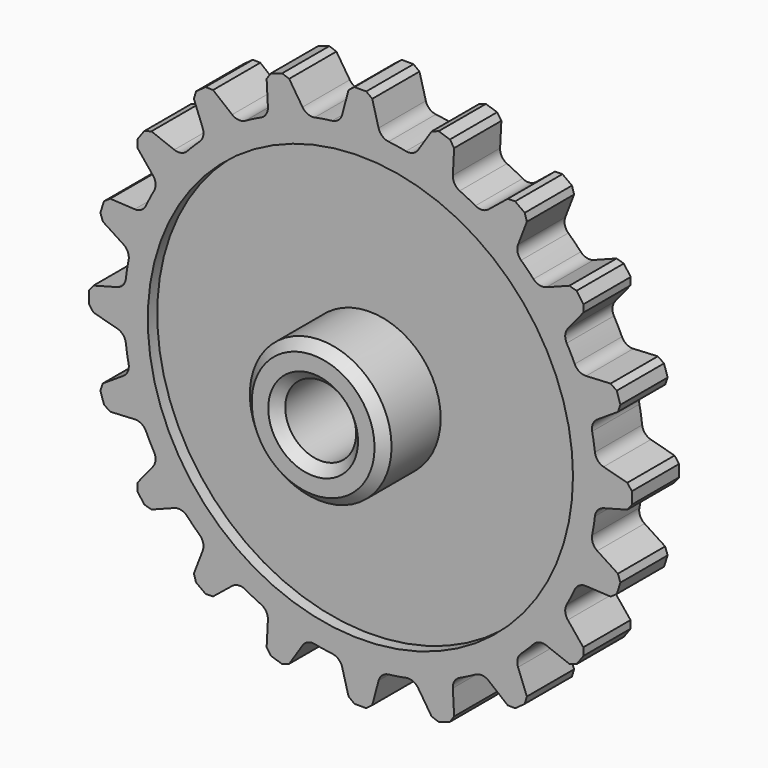
from build123d import *

# Parameters (mm, degrees)
F0_R            = 100
F1_DEPTH        = 25
F3_DEPTH        = 25
F3_COPIES_COUNT = 20
F4_SIZE         = 2
F5_R            = 5
F6_R            = 90
F7_DEPTH        = 5
F8_R            = 30
F9_DEPTH        = 30
F10_R           = 15
F11_DEPTH       = 50.001
F12_SIZE        = 4


# Not quite as in the source:
# - a pattern or mirror of a feature is missing from the dataset's text; its kind, count and spacing are read off the source's solid


with BuildPart() as f1:
    # F0 (on Front) → F1 (new body)
    with BuildSketch(Plane.XZ):
        Circle(F0_R)
    extrude(amount=F1_DEPTH)

    # F2 (on Front) → F3 (join)
    with BuildSketch(Plane.XZ):
        Polygon((-4.5, 114.9222565244), (-8.5976231221, 99.6297188426), (8.5976231221, 99.6297188426), (4.5, 114.9222565244), align=None)
    f3 = extrude(amount=F3_DEPTH)

    # F3_copies: F3 ×20 about axis
    f3_copies_axis = Axis((0, 0, 0), (0, 1, 0))
    for i in range(1, F3_COPIES_COUNT):
        add(f3.rotate(f3_copies_axis, i * 360 / F3_COPIES_COUNT))

    # F4
    f4_edges = [f1.edges().sort_by_distance(p)[0] for p in [
        (4.5, -12.5, 114.922257),
        (-4.5, -12.5, 114.922257),
        (-31.233176, -12.5, 110.688137),
        (110.688137, -12.5, 31.233176),
        (114.922257, -12.5, 4.5),
        (114.922257, -12.5, -4.5),
        (110.688137, -12.5, -31.233176),
        (107.906984, -12.5, -39.792685),
        (95.619092, -12.5, -63.909031),
        (90.329025, -12.5, -71.190184),
        (71.190184, -12.5, -90.329025),
        (63.909031, -12.5, -95.619092),
        (39.792685, -12.5, -107.906984),
        (31.233176, -12.5, -110.688137),
        (4.5, -12.5, -114.922257),
        (-4.5, -12.5, -114.922257),
        (-31.233176, -12.5, -110.688137),
        (-39.792685, -12.5, -107.906984),
        (-63.909031, -12.5, -95.619092),
        (-71.190184, -12.5, -90.329025),
        (-90.329025, -12.5, -71.190184),
        (-95.619092, -12.5, -63.909031),
        (-107.906984, -12.5, -39.792685),
        (-110.688137, -12.5, -31.233176),
        (-114.922257, -12.5, -4.5),
        (-114.922257, -12.5, 4.5),
        (-110.688137, -12.5, 31.233176),
        (-107.906984, -12.5, 39.792685),
        (-95.619092, -12.5, 63.909031),
        (-90.329025, -12.5, 71.190184),
        (-71.190184, -12.5, 90.329025),
        (-63.909031, -12.5, 95.619092),
        (31.233176, -12.5, 110.688137),
        (39.792685, -12.5, 107.906984),
        (63.909031, -12.5, 95.619092),
        (71.190184, -12.5, 90.329025),
        (90.329025, -12.5, 71.190184),
        (95.619092, -12.5, 63.909031),
        (107.906984, -12.5, 39.792685),
        (-39.792685, -12.5, 107.906984),
    ]]
    chamfer(f4_edges, length=F4_SIZE)

    # F5
    f5_edges = [f1.edges().sort_by_distance(p)[0] for p in [
        (8.597623, -12.5, 99.629719),
        (-8.597623, -12.5, 99.629719),
        (97.410305, -12.5, 22.610451),
        (99.629719, -12.5, 8.597623),
        (92.096682, -12.5, 38.964102),
        (85.655692, -12.5, 51.605256),
        (99.629719, -12.5, -8.597623),
        (97.410305, -12.5, -22.610451),
        (75.54858, -12.5, 65.516503),
        (65.516503, -12.5, 75.54858),
        (92.096682, -12.5, -38.964102),
        (85.655692, -12.5, -51.605256),
        (51.605256, -12.5, 85.655692),
        (38.964102, -12.5, 92.096682),
        (75.54858, -12.5, -65.516503),
        (65.516503, -12.5, -75.54858),
        (22.610451, -12.5, 97.410305),
        (51.605256, -12.5, -85.655692),
        (38.964102, -12.5, -92.096682),
        (-22.610451, -12.5, 97.410305),
        (22.610451, -12.5, -97.410305),
        (8.597623, -12.5, -99.629719),
        (-38.964102, -12.5, 92.096682),
        (-51.605256, -12.5, 85.655692),
        (-8.597623, -12.5, -99.629719),
        (-22.610451, -12.5, -97.410305),
        (-65.516503, -12.5, 75.54858),
        (-75.54858, -12.5, 65.516503),
        (-38.964102, -12.5, -92.096682),
        (-51.605256, -12.5, -85.655692),
        (-85.655692, -12.5, 51.605256),
        (-92.096682, -12.5, 38.964102),
        (-65.516503, -12.5, -75.54858),
        (-75.54858, -12.5, -65.516503),
        (-97.410305, -12.5, 22.610451),
        (-99.629719, -12.5, 8.597623),
        (-85.655692, -12.5, -51.605256),
        (-92.096682, -12.5, -38.964102),
        (-99.629719, -12.5, -8.597623),
        (-97.410305, -12.5, -22.610451),
    ]]
    fillet(f5_edges, radius=F5_R)

    # F6 (on face) → F7 (cut)
    with BuildSketch(Plane.XZ.offset(25)):
        Circle(F6_R)
    extrude(amount=-F7_DEPTH, mode=Mode.SUBTRACT)

    # F8 (on face) → F9 (join)
    with BuildSketch(Plane.XZ.offset(20)):
        Circle(F8_R)
    extrude(amount=F9_DEPTH)

    # F10 (on face) → F11 (cut, through all)
    with BuildSketch(Plane.XZ.offset(50)):
        Circle(F10_R)
    extrude(amount=-F11_DEPTH, mode=Mode.SUBTRACT)

    # F12
    f12_edges = [f1.edges().sort_by_distance(p)[0] for p in [
        (-30, -50, 0),
        (-15, -50, 0),
        (15, -25, 0),
        (-15, 0, 0),
    ]]
    chamfer(f12_edges, length=F12_SIZE)


solid = f1.part
